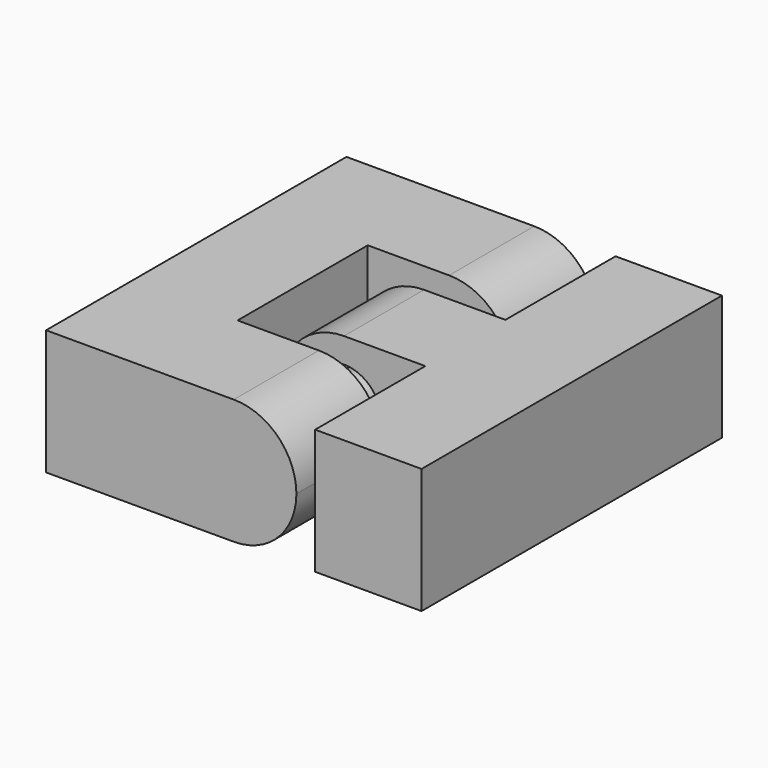
from build123d import *

# Parameters (mm, degrees)
F0_W      = 50.8
F0_H      = 25.4
F1_DEPTH  = 76.2
F2_R      = 12.69999
F3_W      = 28.8026324581
F3_H      = 33.02
F3_W_2    = 16.51001
F4_DEPTH  = 25.4
F5_R      = 5.08
F6_DEPTH  = 34.2138
F7_W      = 50.8
F7_H      = 25.4
F8_DEPTH  = 76.2
F9_W      = 29.21
F9_H      = 27.94
F10_DEPTH = 25.4
F11_R     = 12.69999
F12_R     = 7.62
F13_DEPTH = 25.4


# Not quite as in the source:
# - a fillet or chamfer is up to 0.001 mm smaller than in the source, because OpenCascade refuses the exact size


with BuildPart() as f1:
    # F0 (on Front) → F1 (new body)
    with BuildSketch(Plane.XZ):
        with Locations((12.7, 0)):
            Rectangle(F0_W, F0_H)
    extrude(amount=-F1_DEPTH)

    # F2 (radius 12.7 in the source; OpenCascade refuses exactly that, so slightly less here)
    f2_edges = [f1.edges().sort_by_distance(p)[0] for p in [
        (38.1, 38.1, 12.7),
        (38.1, 38.1, -12.7),
    ]]
    fillet(f2_edges, radius=F2_R)

    # F3 (on face) → F4 (cut)
    with BuildSketch(Plane.XY.offset(12.7)):
        with Locations((39.8013262291, 38.1)):
            Rectangle(F3_W, F3_H)
        with Locations((17.145005, 38.1)):
            Rectangle(F3_W_2, F3_H)
    extrude(amount=-F4_DEPTH, mode=Mode.SUBTRACT)

    # F5 (on face) → F6 (join)
    with BuildSketch(Plane(origin=(0, 21.59, 0), x_dir=(-1, 0, 0), z_dir=(0, 1, 0))):
        with Locations((-25.4, 0)):
            Circle(F5_R)
    extrude(amount=F6_DEPTH)


with BuildPart() as f8:
    # F7 (on Front) → F8 (new body)
    with BuildSketch(Plane.XZ):
        with Locations((38.1, 0)):
            Rectangle(F7_W, F7_H)
    extrude(amount=-F8_DEPTH)

    # F9 (on face) → F10 (cut)
    with BuildSketch(Plane.XY.offset(12.7)):
        with Locations((27.305, 62.23)):
            Rectangle(F9_W, F9_H)
        Polygon((41.91, 76.2), (41.91, 78.74), (-8.89, 78.74), (-8.89, -2.54), (41.91, -2.54), (41.91, 0), (12.7, 0), (12.7, 27.94), (3.81, 27.94), (3.81, 48.26), (12.7, 48.26), (12.7, 76.2), align=None)
        with Locations((27.305, 13.97)):
            Rectangle(F9_W, F9_H)
    extrude(amount=-F10_DEPTH, mode=Mode.SUBTRACT)

    # F11 (radius 12.7 in the source; OpenCascade refuses exactly that, so slightly less here)
    f11_edges = [f8.edges().sort_by_distance(p)[0] for p in [
        (12.7, 38.1, 12.7),
        (12.7, 38.1, -12.7),
    ]]
    fillet(f11_edges, radius=F11_R)

    # F12 (on face) → F13 (cut)
    with BuildSketch(Plane(origin=(0, 48.26, 0), x_dir=(-1, 0, 0), z_dir=(0, 1, 0))):
        with Locations((-25.4, 0)):
            Circle(F12_R)
    extrude(amount=-F13_DEPTH, mode=Mode.SUBTRACT)


solid = Compound([f1.part, f8.part])
